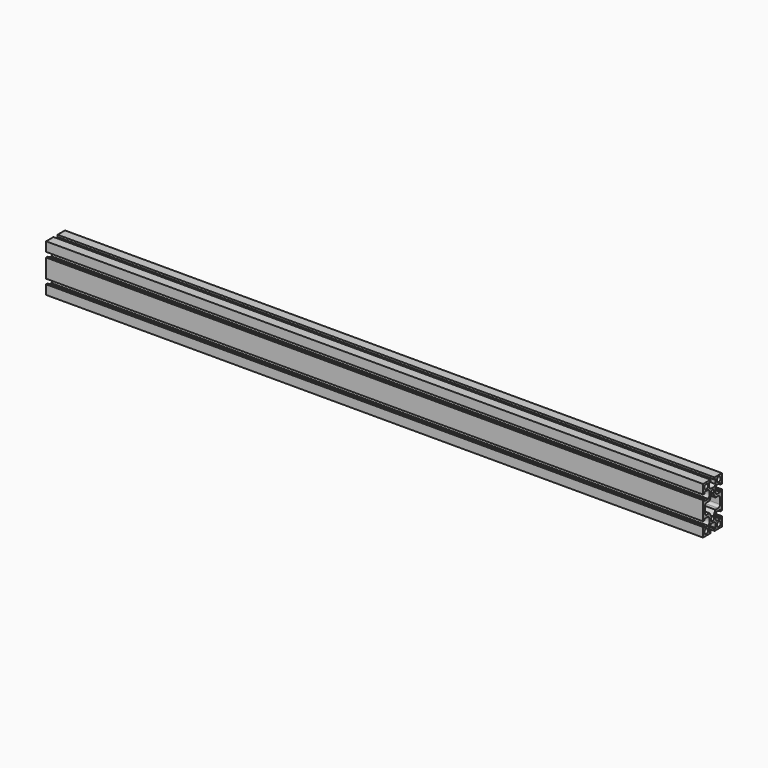
from build123d import *

# Parameters (mm, degrees)
F0_R     = 3
F1_DEPTH = 835


# Not quite as in the source:
# - ends of sketch curves that miss each other by under 0.0002 mm in the source are joined


with BuildPart() as f1:
    # F0 (on Right) → F1 (new body)
    with BuildSketch(Plane.YZ):
        with BuildLine():
            Line((12.5, -11.85), (15, -11.85))
            Line((15, -11.85), (15, 11.85))
            Line((15, 11.85), (12.5, 11.85))
            Line((12.5, 11.85), (12.5, 9.85))
            Line((12.5, 9.85), (6.547707, 9.85))
            ThreePointArc((6.5477069495, 9.8499999523), (4.5, 15), (6.5477069495, 20.1500000477))
            Line((6.547707, 20.15), (12.5, 20.15))
            Line((12.5, 20.15), (12.5, 18.15))
            Line((12.5, 18.15), (15, 18.15))
            Line((15, 18.15), (15, 30))
            Line((15, 30), (3.15, 30))
            Line((3.15, 30), (3.15, 27.5))
            Line((3.15, 27.5), (5.15, 27.5))
            Line((5.15, 27.5), (5.15, 21.547707))
            ThreePointArc((5.1500000477, 21.5477069495), (0, 19.5), (-5.1500000477, 21.5477069495))
            Line((-5.15, 21.547707), (-5.15, 27.5))
            Line((-5.15, 27.5), (-3.15, 27.5))
            Line((-3.15, 27.5), (-3.15, 30))
            Line((-3.15, 30), (-15, 30))
            Line((-15, 30), (-15, 18.15))
            Line((-15, 18.15), (-12.5, 18.15))
            Line((-12.5, 18.15), (-12.5, 20.15))
            Line((-12.5, 20.15), (-6.547707, 20.15))
            ThreePointArc((-6.5477069495, 20.1500000477), (-4.5, 15), (-6.5477069495, 9.8499999523))
            Line((-6.547707, 9.85), (-12.5, 9.85))
            Line((-12.5, 9.85), (-12.5, 11.85))
            Line((-12.5, 11.85), (-15, 11.85))
            Line((-15, 11.85), (-15, -11.85))
            Line((-15, -11.85), (-12.5, -11.85))
            Line((-12.5, -11.85), (-12.5, -9.85))
            Line((-12.5, -9.85), (-6.547707, -9.85))
            ThreePointArc((-6.5477069495, -9.8499999523), (-4.5, -15), (-6.5477069495, -20.1500000477))
            Line((-6.547707, -20.15), (-12.5, -20.15))
            Line((-12.5, -20.15), (-12.5, -18.15))
            Line((-12.5, -18.15), (-15, -18.15))
            Line((-15, -18.15), (-15, -30))
            Line((-15, -30), (-3.15, -30))
            Line((-3.15, -30), (-3.15, -27.5))
            Line((-3.15, -27.5), (-5.15, -27.5))
            Line((-5.15, -27.5), (-5.15, -21.547707))
            ThreePointArc((-5.1500000477, -21.5477069495), (0, -19.5), (5.1500000477, -21.5477069495))
            Line((5.15, -21.547707), (5.15, -27.5))
            Line((5.15, -27.5), (3.15, -27.5))
            Line((3.15, -27.5), (3.15, -30))
            Line((3.15, -30), (15, -30))
            Line((15, -30), (15, -18.15))
            Line((15, -18.15), (12.5, -18.15))
            Line((12.5, -18.15), (12.5, -20.15))
            Line((12.5, -20.15), (6.547707, -20.15))
            ThreePointArc((6.5477069495, -20.1500000477), (4.5, -15), (6.5477069495, -9.8499999523))
            Line((6.547707, -9.85), (12.5, -9.85))
            Line((12.5, -9.85), (12.5, -11.85))
        make_face()
        with Locations((-10, -25)):
            Circle(F0_R, mode=Mode.SUBTRACT)
        with Locations((10, -25)):
            Circle(F0_R, mode=Mode.SUBTRACT)
        with Locations((-10, 25)):
            Circle(F0_R, mode=Mode.SUBTRACT)
        with BuildLine():
            ThreePointArc((-12, 3.85), (-11.1213203436, 5.9713203436), (-9, 6.85))
            Line((-9, 6.85), (-4.705405, 6.85))
            Line((-4.705405, 6.85), (-1.25, 12.834936))
            ThreePointArc((-1.25, 12.834936), (0, 17.5), (1.2499997876, 12.8349363679))
            Line((1.2499997876, 12.8349363679), (4.705405, 6.85))
            Line((4.705405, 6.85), (9, 6.85))
            ThreePointArc((9, 6.85), (11.1213203436, 5.9713203436), (12, 3.85))
            Line((12, 3.85), (12, -3.85))
            ThreePointArc((12, -3.85), (11.1213203436, -5.9713203436), (9, -6.85))
            Line((9, -6.85), (4.705405, -6.85))
            Line((4.705405, -6.85), (1.25, -12.834937))
            ThreePointArc((1.25, -12.834937), (0, -17.5), (-1.2500002206, -12.8349366179))
            Line((-1.2500002206, -12.8349366179), (-4.705405, -6.85))
            Line((-4.705405, -6.85), (-9, -6.85))
            ThreePointArc((-9, -6.85), (-11.1213203436, -5.9713203436), (-12, -3.85))
            Line((-12, -3.85), (-12, 3.85))
        make_face(mode=Mode.SUBTRACT)
        with Locations((10, 25)):
            Circle(F0_R, mode=Mode.SUBTRACT)
    extrude(amount=F1_DEPTH)


solid = f1.part
